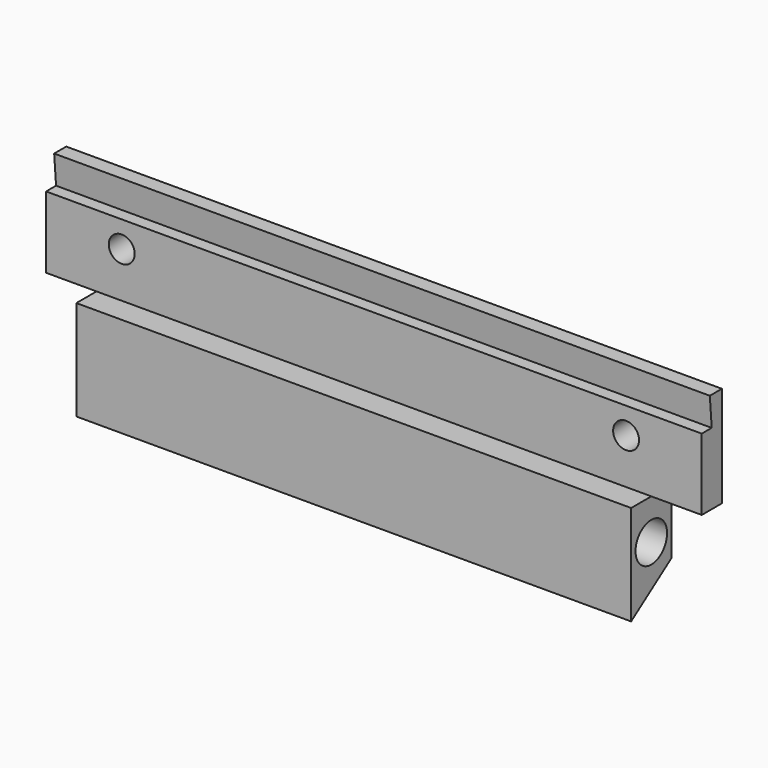
from build123d import *

# Parameters (mm, degrees)
F0_W         = 165.1
F0_H         = 38.1
F1_DEPTH     = 12.7
F3_DEPTH     = 165.101
F4_W         = 165.1
F4_H         = 12.7
F5_DEPTH     = 12.7
F7_D         = 6.5278
F9_W         = 12.7
F9_H         = 25.4
F10_DEPTH    = 12.701
F11_D        = 9.9314
F12_T1_DEPTH = 207.1510236039


# Not quite as in the source:
# - a fillet or chamfer that OpenCascade refuses, or shapes differently, is made with other operations: its cross-section is extruded or revolved along the edge and cut away or added


with BuildPart() as f1:
    # F0 (on Front) → F1 (new body)
    with BuildSketch(Plane.XZ):
        with Locations((82.55, 19.05)):
            Rectangle(F0_W, F0_H)
    extrude(amount=F1_DEPTH)

    # F2 (on face) → F3 (cut, through all)
    with BuildSketch(Plane.YZ.offset(165.1)):
        Polygon((-6.35, 12.7), (-6.35, 30.734), (-3.2131, 30.734), (-3.81, 38.1), (-8.89, 38.1), (-12.7, 38.1), (-12.7, 27.7622), (-12.7, 12.7), align=None)
    extrude(amount=-F3_DEPTH, mode=Mode.SUBTRACT)

    # F4 (on face) → F5 (join)
    with BuildSketch(Plane.XZ.offset(12.7)):
        with Locations((82.55, -6.35)):
            Rectangle(F4_W, F4_H)
    extrude(amount=-F5_DEPTH)

    # F7 (through all)
    with Locations(Plane.XZ.offset(6.35)):
        with Locations((19.05, 24.13), (146.05, 24.13)):
            Hole(F7_D / 2)

    # F9 (on face) → F10 (cut, through all)
    with BuildSketch(Plane.XZ.offset(12.7)):
        with Locations((6.35, 0)):
            Rectangle(F9_W, F9_H)
        with Locations((158.75, 0)):
            Rectangle(F9_W, F9_H)
    extrude(amount=-F10_DEPTH, mode=Mode.SUBTRACT)

    # F11 (through all)
    with Locations(Plane(origin=(0, 0, 0), x_dir=(0, -1, 0), z_dir=(-1, 0, 0))):
        with Locations((6.35, 2.54)):
            Hole(F11_D / 2)

    # F12: chamfer of 9.144 x 13.0589853736 on 1 edges, made by hand

    # F12_s2 → F12_t1 (cut)
    with BuildSketch(Plane.YZ.offset(-21.025511802)):
        Polygon((0, -3.556), (-13.0589853736, -12.7), (0, -12.7), align=None)
    extrude(amount=F12_T1_DEPTH, mode=Mode.SUBTRACT)


solid = f1.part
